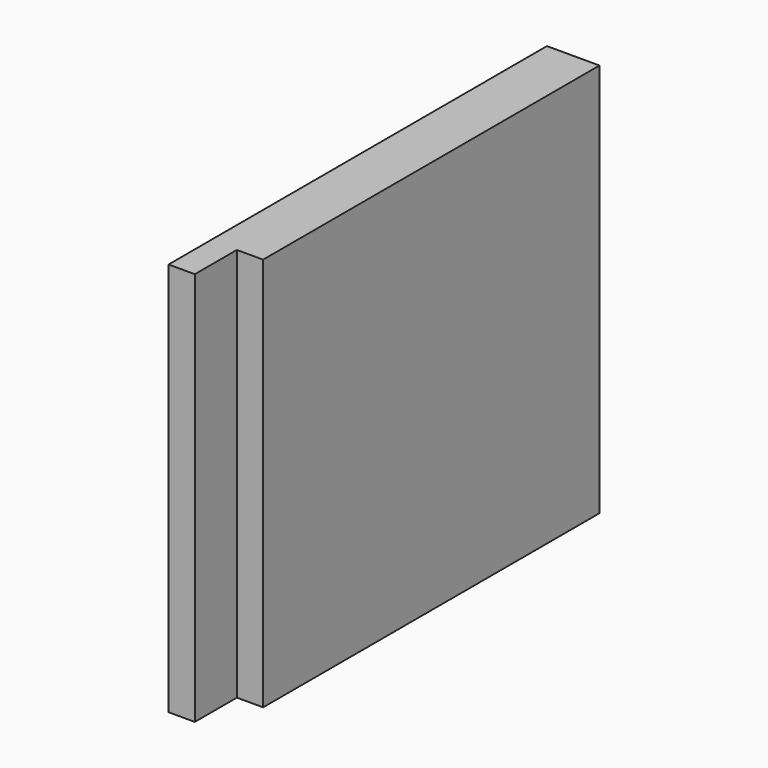
from build123d import *

# Parameters (mm, degrees)
F0_W     = 180
F0_H     = 150
F1_DEPTH = 20
F2_W     = 10
F2_H     = 150
F3_DEPTH = 20


# Not quite as in the source:
# - the program builds the solid bodies; features that only make, move or delete a surface that nothing else refers to are left out


with BuildPart() as f1:
    # F0 (on Right) → F1 (new body)
    with BuildSketch(Plane.YZ):
        with Locations((6.5838837624, 31.891247511)):
            Rectangle(F0_W, F0_H)
    extrude(amount=F1_DEPTH)

    # F2 (on face) → F3 (cut)
    with BuildSketch(Plane.XZ.offset(83.4161162376)):
        with Locations((15, 31.891247511)):
            Rectangle(F2_W, F2_H)
    extrude(amount=-F3_DEPTH, mode=Mode.SUBTRACT)


solid = f1.part
